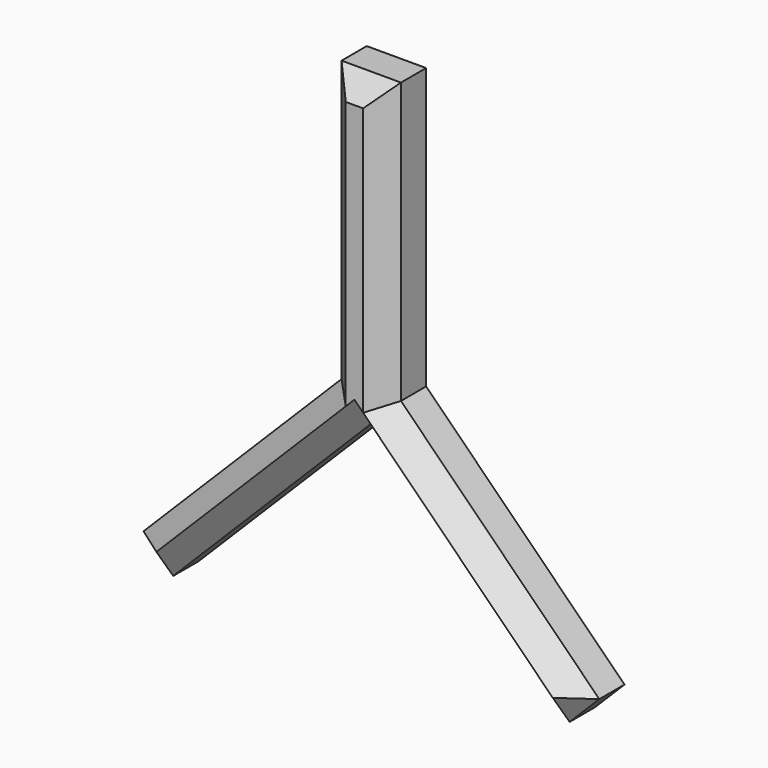
from build123d import *

# Parameters (mm, degrees)
F1_DEPTH = 12.7
F2_SIZE  = 5.07999


# Not quite as in the source:
# - a fillet or chamfer is up to 0.001 mm smaller than in the source, because OpenCascade refuses the exact size


with BuildPart() as f1:
    # F0 (on Front) → F1 (new body)
    with BuildSketch(Plane.XZ):
        Polygon((-7.1858047352, 75.0022197947), (-7.1858047352, 7.1842197947), (-55.1002257696, -40.8236010231), (-47.909149441, -48.0009279096), (0, 0), (48.0004344931, -47.9086569679), (55.1777613797, -40.7175806394), (7.1841965553, 7.1842197947), (7.1841965553, 75.0022197947), align=None)
    extrude(amount=F1_DEPTH)

    # F2 (size 5.08 in the source; OpenCascade refuses exactly that, so slightly less here)
    f2_edges = [f1.edges().sort_by_distance(p)[0] for p in [
        (7.184197, -12.7, 41.09322),
        (-0.000804, -12.7, 75.00222),
        (-7.185805, -12.7, 41.09322),
        (-31.143015, -12.7, -16.819691),
        (-51.504688, -12.7, -44.412264),
        (-23.954575, -12.7, -24.000464),
        (24.000217, -12.7, -23.954328),
        (51.589098, -12.7, -44.313119),
        (31.180979, -12.7, -16.76668),
    ]]
    chamfer(f2_edges, length=F2_SIZE)


solid = f1.part
